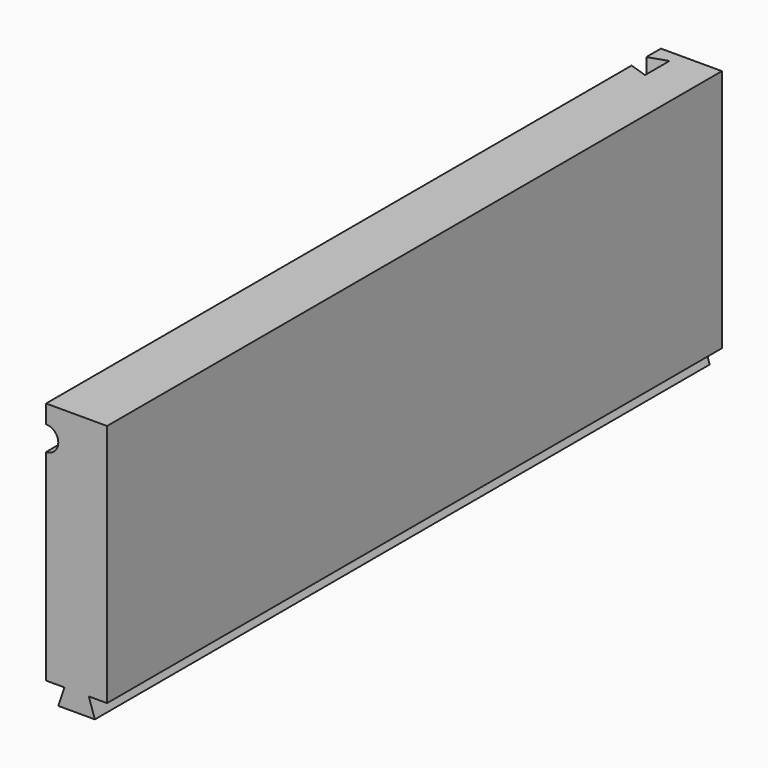
from build123d import *

# Parameters (mm, degrees)
F0_W     = 63
F0_H     = 21.5
F1_DEPTH = 5
F3_DEPTH = 63.001
F4_DEPTH = 58
F6_DEPTH = 20


# Not quite as in the source:
# - a feature names something its author has since deleted; it is built from what else it names


with BuildPart() as f1:
    # F0 (on Right) → F1 (new body)
    with BuildSketch(Plane.YZ):
        Rectangle(F0_W, F0_H)
    extrude(amount=F1_DEPTH)

    # F2 (on face) → F3 (cut, through all)
    with BuildSketch(Plane.XZ.offset(31.5)):
        Polygon((1.5, -9.25), (0, -9.25), (0, -10.75), (1, -10.75), align=None)
        Polygon((3.5, -9.25), (4, -10.75), (5, -10.75), (5, -9.25), align=None)
    extrude(amount=-F3_DEPTH, mode=Mode.SUBTRACT)

    # F2 (on face) → F4 (cut)
    with BuildSketch(Plane.XZ.offset(31.5)):
        with BuildLine():
            Line((0, 9.25), (0, 7.25))
            ThreePointArc((0, 7.25), (1, 8.25), (0, 9.25))
        make_face()
    extrude(amount=-F4_DEPTH, mode=Mode.SUBTRACT)

    # F5 (on face) → F6 (cut, through all)
    with BuildSketch(Plane.XY.offset(10.75)):
        Polygon((1.5, 30.5), (0, 30), (0, 28.5), (1.5, 28), align=None)
    extrude(amount=-F6_DEPTH, mode=Mode.SUBTRACT)


solid = f1.part
